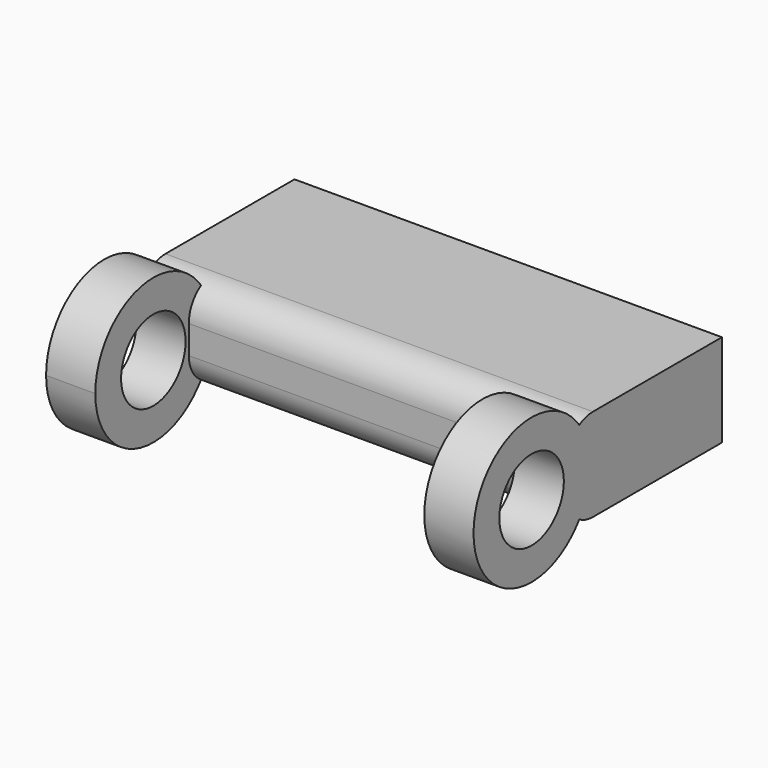
from build123d import *

# Parameters (mm, degrees)
F0_W         = 53
F0_H         = 11.5
F0_W_2       = 48
F0_H_2       = 6.5
F1_DEPTH     = 4
F2_DEPTH     = 20
F4_R         = 5
F5_DEPTH     = 6.1
F3_R         = 5
F6_DEPTH     = 6.1
F7_T4_DEPTH  = 50.8
F7_S5_R      = 9
F7_T6_DEPTH  = 27
F7_T11_DEPTH = 40.8
F7_S12_R     = 9
F7_T13_DEPTH = 22
F7_T17_DEPTH = 40.8
F7_S18_R     = 9
F7_T19_DEPTH = 22
F7_T23_DEPTH = 50.8
F7_S24_R     = 9
F7_T25_DEPTH = 27
F7_T30_DEPTH = 50.8
F7_S31_R     = 9
F7_T32_DEPTH = 27
F7_T37_DEPTH = 40.8
F7_S38_R     = 9
F7_T39_DEPTH = 22
F7_T43_DEPTH = 40.8
F7_S44_R     = 9
F7_T45_DEPTH = 22
F7_T49_DEPTH = 50.8
F7_S50_R     = 9
F7_T51_DEPTH = 27


# Not quite as in the source:
# - a fillet or chamfer that OpenCascade refuses, or shapes differently, is made with other operations: its cross-section is extruded or revolved along the edge and cut away or added


with BuildPart() as f1:
    # F0 (on Front) → F1 (new body)
    with BuildSketch(Plane.XZ):
        Rectangle(F0_W, F0_H)
        Rectangle(F0_W_2, F0_H_2, mode=Mode.SUBTRACT)
        Rectangle(F0_W_2, F0_H_2)
    extrude(amount=F1_DEPTH)

    # F0 (on Front) → F2 (join)
    with BuildSketch(Plane.XZ):
        Rectangle(F0_W, F0_H)
        Rectangle(F0_W_2, F0_H_2, mode=Mode.SUBTRACT)
    extrude(amount=-F2_DEPTH)

    # F4 (on face) → F5 (join)
    with BuildSketch(Plane(origin=(-26.5, 0, 0), x_dir=(0, -1, 0), z_dir=(-1, 0, 0))):
        with BuildLine():
            ThreePointArc((2.576309, -5.75), (12.556696, -8.465023), (18.5, 0))
            ThreePointArc((18.5, 0), (12.556696, 8.465023), (2.576309, 5.75))
            Line((2.576309, 5.75), (4, 5.75))
            Line((4, 5.75), (4, -5.75))
            Line((4, -5.75), (2.576309, -5.75))
        make_face()
        with Locations((9.5, 0)):
            Circle(F4_R, mode=Mode.SUBTRACT)
    extrude(amount=-F5_DEPTH)

    # F3 (on face) → F6 (join)
    with BuildSketch(Plane.YZ.offset(26.5)):
        with BuildLine():
            Line((-4, 5.75), (-2.576309, 5.75))
            ThreePointArc((-2.576309, 5.75), (-18.5, 0), (-2.576309, -5.75))
            Line((-2.576309, -5.75), (-4, -5.75))
            Line((-4, -5.75), (-4, 5.75))
        make_face()
        with Locations((-9.5, 0)):
            Circle(F3_R, mode=Mode.SUBTRACT)
    extrude(amount=-F6_DEPTH)

    # F7: fillet of radius 4 on 2 edges, made by hand


with BuildPart() as f7_tool2:
    # F7_s3 → F7_t4 (new body)
    with BuildSketch(Plane.YZ.offset(30.4)):
        with BuildLine():
            ThreePointArc((0, 5.75), (-2.828427, 4.578427), (-4, 1.75))
            Line((-4, 1.75), (-4, 5.75))
            Line((-4, 5.75), (0, 5.75))
        make_face()
    extrude(amount=-F7_T4_DEPTH)

    # F7_s5 → F7_t6 (cut, symmetric)
    with BuildSketch(Plane.YZ.offset(5)):
        with Locations((-9.5, 0)):
            Circle(F7_S5_R)
    extrude(amount=F7_T6_DEPTH, both=True, mode=Mode.SUBTRACT)

    split(bisect_by=Plane.YZ.offset(20.4), keep=Keep.TOP)


with BuildPart() as f1_1:
    add(f1.part)

    # F7_t1: cut F7_tool2
    add(f7_tool2.part, mode=Mode.SUBTRACT)


with BuildPart() as f7_tool9:
    # F7_s10 → F7_t11 (new body)
    with BuildSketch(Plane.YZ.offset(20.4)):
        with BuildLine():
            ThreePointArc((0, 5.75), (-2.828427, 4.578427), (-4, 1.75))
            Line((-4, 1.75), (-4, 5.75))
            Line((-4, 5.75), (0, 5.75))
        make_face()
    extrude(amount=-F7_T11_DEPTH)

    # F7_s12 → F7_t13 (cut, symmetric)
    with BuildSketch(Plane.YZ):
        with Locations((-9.5, 0)):
            Circle(F7_S12_R)
    extrude(amount=F7_T13_DEPTH, both=True, mode=Mode.SUBTRACT)


with BuildPart() as f1_2:
    add(f1_1.part)

    # F7_t8: cut F7_tool9
    add(f7_tool9.part, mode=Mode.SUBTRACT)


with BuildPart() as f7_tool15:
    # F7_s16 → F7_t17 (new body)
    with BuildSketch(Plane.YZ.offset(20.4)):
        with BuildLine():
            ThreePointArc((0, 5.75), (-2.828427, 4.578427), (-4, 1.75))
            Line((-4, 1.75), (-4, 5.75))
            Line((-4, 5.75), (0, 5.75))
        make_face()
    extrude(amount=-F7_T17_DEPTH)

    # F7_s18 → F7_t19 (intersect, symmetric)
    with BuildSketch(Plane.YZ):
        with Locations((-9.5, 0)):
            Circle(F7_S18_R)
    extrude(amount=F7_T19_DEPTH, both=True, mode=Mode.INTERSECT)


with BuildPart() as f1_3:
    add(f1_2.part)

    # F7_t14: cut F7_tool15
    add(f7_tool15.part, mode=Mode.SUBTRACT)


with BuildPart() as f7_tool21:
    # F7_s22 → F7_t23 (new body)
    with BuildSketch(Plane.YZ.offset(20.4)):
        with BuildLine():
            ThreePointArc((0, 5.75), (-2.828427, 4.578427), (-4, 1.75))
            Line((-4, 1.75), (-4, 5.75))
            Line((-4, 5.75), (0, 5.75))
        make_face()
    extrude(amount=-F7_T23_DEPTH)

    # F7_s24 → F7_t25 (cut, symmetric)
    with BuildSketch(Plane.YZ.offset(-5)):
        with Locations((-9.5, 0)):
            Circle(F7_S24_R)
    extrude(amount=F7_T25_DEPTH, both=True, mode=Mode.SUBTRACT)

    split(bisect_by=Plane.YZ.offset(-20.4), keep=Keep.BOTTOM)


with BuildPart() as f1_4:
    add(f1_3.part)

    # F7_t20: cut F7_tool21
    add(f7_tool21.part, mode=Mode.SUBTRACT)


with BuildPart() as f7_tool28:
    # F7_s29 → F7_t30 (new body)
    with BuildSketch(Plane.YZ.offset(-30.4)):
        with BuildLine():
            ThreePointArc((0, -5.75), (-2.828427, -4.578427), (-4, -1.75))
            Line((-4, -1.75), (-4, -5.75))
            Line((-4, -5.75), (0, -5.75))
        make_face()
    extrude(amount=F7_T30_DEPTH)

    # F7_s31 → F7_t32 (cut, symmetric)
    with BuildSketch(Plane.YZ.offset(-5)):
        with Locations((-9.5, 0)):
            Circle(F7_S31_R)
    extrude(amount=F7_T32_DEPTH, both=True, mode=Mode.SUBTRACT)

    split(bisect_by=Plane.YZ.offset(-20.4), keep=Keep.BOTTOM)


with BuildPart() as f1_5:
    add(f1_4.part)

    # F7_t27: cut F7_tool28
    add(f7_tool28.part, mode=Mode.SUBTRACT)


with BuildPart() as f7_tool35:
    # F7_s36 → F7_t37 (new body)
    with BuildSketch(Plane.YZ.offset(-20.4)):
        with BuildLine():
            ThreePointArc((0, -5.75), (-2.828427, -4.578427), (-4, -1.75))
            Line((-4, -1.75), (-4, -5.75))
            Line((-4, -5.75), (0, -5.75))
        make_face()
    extrude(amount=F7_T37_DEPTH)

    # F7_s38 → F7_t39 (cut, symmetric)
    with BuildSketch(Plane.YZ):
        with Locations((-9.5, 0)):
            Circle(F7_S38_R)
    extrude(amount=F7_T39_DEPTH, both=True, mode=Mode.SUBTRACT)


with BuildPart() as f1_6:
    add(f1_5.part)

    # F7_t34: cut F7_tool35
    add(f7_tool35.part, mode=Mode.SUBTRACT)


with BuildPart() as f7_tool41:
    # F7_s42 → F7_t43 (new body)
    with BuildSketch(Plane.YZ.offset(-20.4)):
        with BuildLine():
            ThreePointArc((0, -5.75), (-2.828427, -4.578427), (-4, -1.75))
            Line((-4, -1.75), (-4, -5.75))
            Line((-4, -5.75), (0, -5.75))
        make_face()
    extrude(amount=F7_T43_DEPTH)

    # F7_s44 → F7_t45 (intersect, symmetric)
    with BuildSketch(Plane.YZ):
        with Locations((-9.5, 0)):
            Circle(F7_S44_R)
    extrude(amount=F7_T45_DEPTH, both=True, mode=Mode.INTERSECT)


with BuildPart() as f1_7:
    add(f1_6.part)

    # F7_t40: cut F7_tool41
    add(f7_tool41.part, mode=Mode.SUBTRACT)


with BuildPart() as f7_tool47:
    # F7_s48 → F7_t49 (new body)
    with BuildSketch(Plane.YZ.offset(-20.4)):
        with BuildLine():
            ThreePointArc((0, -5.75), (-2.828427, -4.578427), (-4, -1.75))
            Line((-4, -1.75), (-4, -5.75))
            Line((-4, -5.75), (0, -5.75))
        make_face()
    extrude(amount=F7_T49_DEPTH)

    # F7_s50 → F7_t51 (cut, symmetric)
    with BuildSketch(Plane.YZ.offset(5)):
        with Locations((-9.5, 0)):
            Circle(F7_S50_R)
    extrude(amount=F7_T51_DEPTH, both=True, mode=Mode.SUBTRACT)

    split(bisect_by=Plane.YZ.offset(20.4), keep=Keep.TOP)


with BuildPart() as f1_8:
    add(f1_7.part)

    # F7_t46: cut F7_tool47
    add(f7_tool47.part, mode=Mode.SUBTRACT)


solid = f1_8.part
